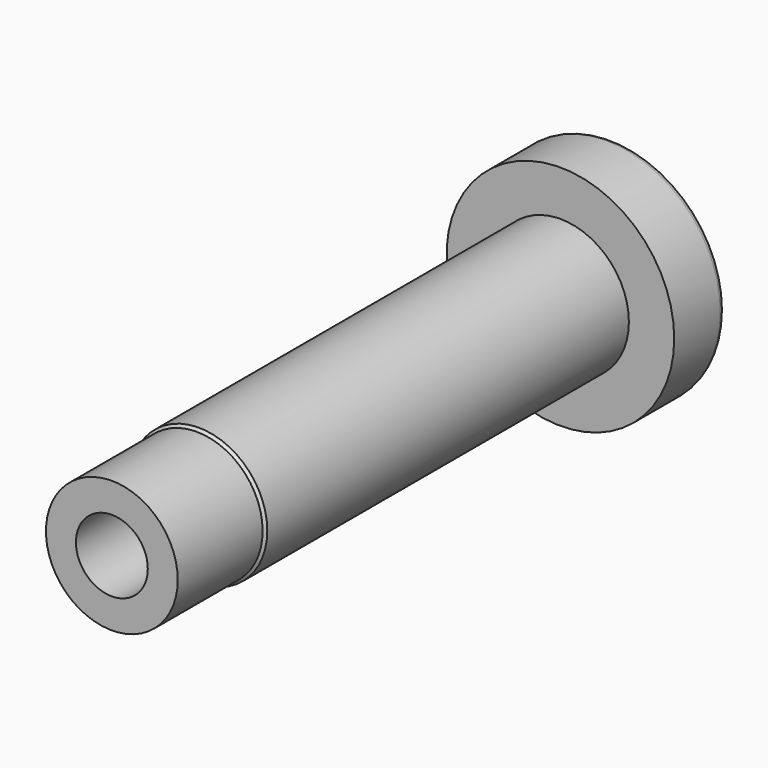
from build123d import *

# Parameters (mm, degrees)
F0_R        = 57.15
F1_DEPTH    = 382.27
F2_R        = 95.004000019
F3_DEPTH    = 53
F4_R        = 5
F5_R        = 55
F5_R_2      = 30
F6_DEPTH    = 85.7
F7_S5_R     = 55
F7_T6_DEPTH = 82


# Not quite as in the source:
# - a fillet or chamfer that OpenCascade refuses, or shapes differently, is made with other operations: its cross-section is extruded or revolved along the edge and cut away or added


with BuildPart() as f1:
    # F0 (on Front) → F1 (new body)
    with BuildSketch(Plane.XZ):
        Circle(F0_R)
    extrude(amount=F1_DEPTH)

    # F2 (on Front) → F3 (join)
    with BuildSketch(Plane.XZ):
        Circle(F2_R)
    extrude(amount=-F3_DEPTH)

    # F4
    f4_edges = [f1.edges().sort_by_distance(p)[0] for p in [
        (-95.004, 53, 0),
    ]]
    fillet(f4_edges, radius=F4_R)

    # F5 (on face) → F6 (join)
    with BuildSketch(Plane.XZ.offset(382.27)):
        Circle(F5_R)
        Circle(F5_R_2, mode=Mode.SUBTRACT)
    extrude(amount=F6_DEPTH)

    # F7: chamfer of 5 on 1 edges, made by hand


with BuildPart() as f7_tool2:
    # F7_s3 → F7_t4 (revolve)
    with BuildSketch(Plane.XY):
        Polygon((57.15, -377.27), (52.15, -382.27), (57.15, -382.27), align=None)
    revolve(axis=Axis((0, -382.27, 0), (0, -1, 0)))

    # F7_s5 → F7_t6 (cut, symmetric)
    with BuildSketch(Plane.XZ.offset(379.8)):
        Circle(F7_S5_R)
    extrude(amount=F7_T6_DEPTH, both=True, mode=Mode.SUBTRACT)


with BuildPart() as f1_1:
    add(f1.part)

    # F7_t1: cut F7_tool2
    add(f7_tool2.part, mode=Mode.SUBTRACT)


solid = f1_1.part
